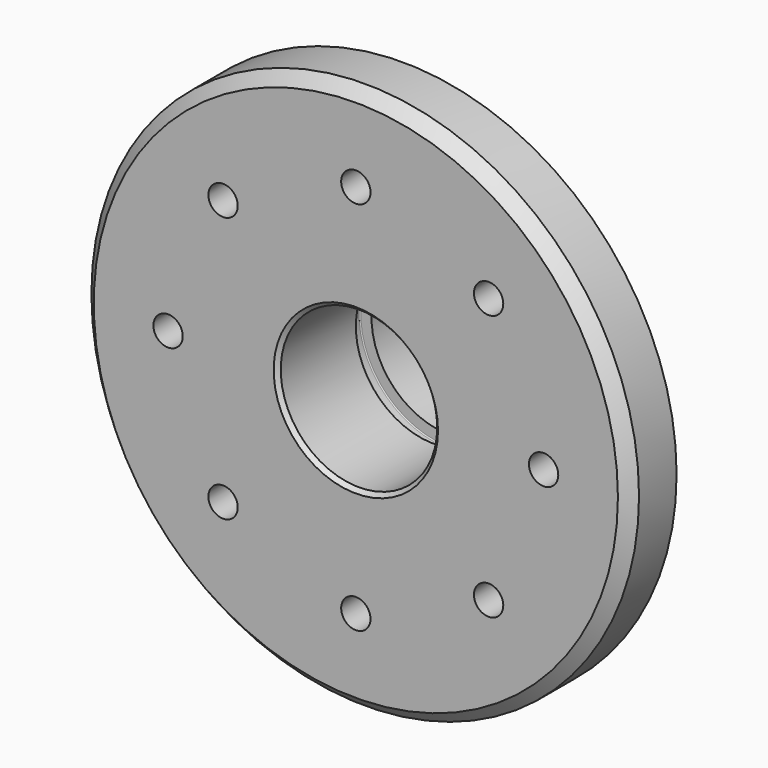
from build123d import *

# Parameters (mm, degrees)
F2_R            = 2.5
F3_R            = 0.25
F4_SIZE         = 1
F5_SIZE         = 3
F7_D            = 7.5
F7_COPIES_COUNT = 8
F8_W            = 5
F8_H            = 12.3844173994
F10_W           = 3.9803426395
F10_H           = 3


# Not quite as in the source:
# - a pattern or mirror of a feature is missing from the dataset's text; its kind, count and spacing are read off the source's solid


with BuildPart() as f1:
    # F0 (on Top) → F1 (revolve)
    with BuildSketch(Plane.XY):
        Polygon((70, 15), (35, 15), (35, 40), (20, 40), (20, 30), (23, 30), (23, 25), (20, 25), (20, 0), (70, 0), align=None)
    revolve(axis=Axis((0, 48.9874315186, 0), (0, 1, 0)))

    # F2
    f2_edges = [f1.edges().sort_by_distance(p)[0] for p in [
        (-35, 15, 0),
    ]]
    fillet(f2_edges, radius=F2_R)

    # F3
    f3_edges = [f1.edges().sort_by_distance(p)[0] for p in [
        (-23, 30, 0),
        (-23, 25, 0),
    ]]
    fillet(f3_edges, radius=F3_R)

    # F4
    f4_edges = [f1.edges().sort_by_distance(p)[0] for p in [
        (-20, 0, 0),
    ]]
    chamfer(f4_edges, length=F4_SIZE)

    # F5
    f5_edges = [f1.edges().sort_by_distance(p)[0] for p in [
        (-70, 0, 0),
    ]]
    chamfer(f5_edges, length=F5_SIZE)

    # F7 (through all)
    with Locations(Plane(origin=(0, 15, 0), x_dir=(-1, 0, 0), z_dir=(0, 1, 0))):
        with Locations((0, -48)):
            f7 = Hole(F7_D / 2)

    # F7_copies: F7 ×8 about axis
    f7_copies_axis = Axis((0, 0, 0), (0, 1, 0))
    for i in range(1, F7_COPIES_COUNT):
        add(f7.rotate(f7_copies_axis, i * 360 / F7_COPIES_COUNT), mode=Mode.SUBTRACT)

    # F8 (on Right) → F9 (revolve, cut)
    with BuildSketch(Plane.YZ):
        with Locations((31.5, 39.1922086997)):
            Rectangle(F8_W, F8_H)
    revolve(axis=Axis((0, 33.8349905132, 0), (0, 1, 0)), mode=Mode.SUBTRACT)

    # F10 (on Right) → F11 (revolve, cut)
    with BuildSketch(Plane.YZ):
        with Locations((40.9901713197, 29.5)):
            Rectangle(F10_W, F10_H)
    revolve(axis=Axis((0, 26.3936025676, 0), (0, 1, 0)), mode=Mode.SUBTRACT)


solid = f1.part
